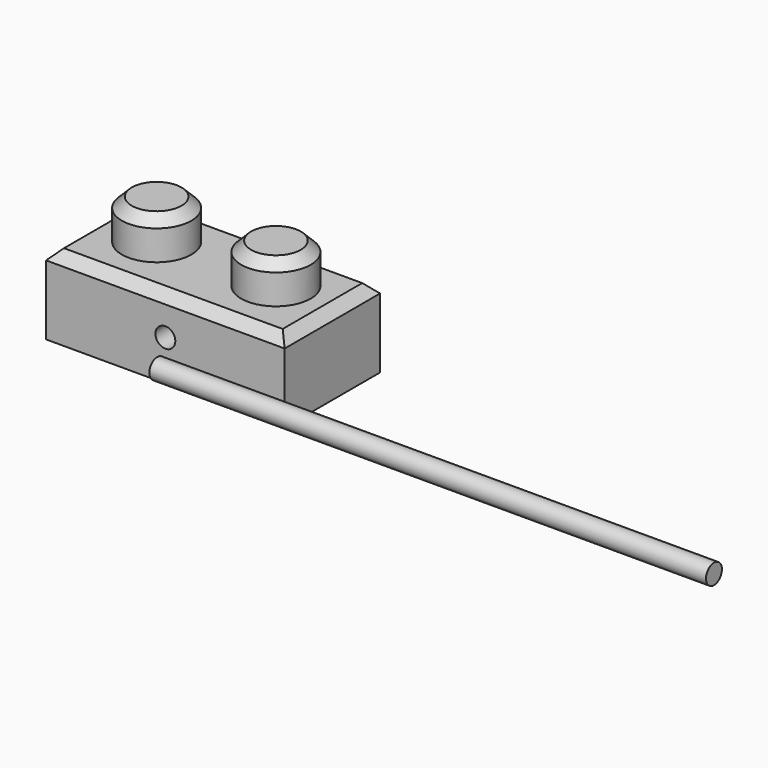
from build123d import *

# Parameters (mm, degrees)
F0_W          = 76.2
F0_H          = 38.1
F1_DEPTH      = 25.4
F2_R          = 11.1125
F3_DEPTH      = 12.7
F4_SIZE2      = 3.175
F4_SIZE       = 3.175
F5_SIZE       = 3.175
F6_T          = 7.9375
F7_R          = 3.175
F8_DEPTH      = 20.3260867754
F8_DEPTH_BACK = 17.7759132246
F9_R          = 3.175
F10_DEPTH     = 177.8


# Not quite as in the source:
# - a shell that OpenCascade refuses in one call is made with other operations: the cavity is built on its own and cut out


with BuildPart() as f1:
    # F0 (on Top) → F1 (new body)
    with BuildSketch(Plane.XY):
        with Locations((-14.6912483396, -1.2750867754)):
            Rectangle(F0_W, F0_H)
    extrude(amount=F1_DEPTH)

    # F2 (on face) → F3 (join)
    with BuildSketch(Plane.XY.offset(25.4)):
        with Locations((-33.7412483396, 0)):
            Circle(F2_R)
        with Locations((4.3587516604, 0)):
            Circle(F2_R)
    extrude(amount=F3_DEPTH)

    # F4
    f4_edges = [f1.edges().sort_by_distance(p)[0] for p in [
        (-14.691248, -20.325087, 25.4),
        (-52.791248, -1.275087, 25.4),
        (-14.691248, 17.774913, 25.4),
        (23.408752, -1.275087, 25.4),
    ]]
    chamfer(f4_edges, length=F4_SIZE, length2=F4_SIZE2)

    # F5
    f5_edges = [f1.edges().sort_by_distance(p)[0] for p in [
        (-44.853748, 0, 38.1),
        (-6.753748, 0, 38.1),
    ]]
    chamfer(f5_edges, length=F5_SIZE)

    # F6: shell of thickness 7.9375, made by hand


with BuildPart() as f6_core1:
    # F6_t2: copy of F1
    add(f1.part)

    # the walls: a layer under each face that stays
    f6_faces = [f6_core1.faces().sort_by_distance(p)[0] for p in [
        (-44.8537483396, 0, 30.1625),
        (-43.2662483396, 0, 36.5125),
        (-14.6912483396, -1.2750867754, 25.4),
        (-33.7412483396, 0, 38.1),
        (-14.6912483396, -18.7375867754, 23.8125),
        (-51.2037483396, -1.2750867754, 23.8125),
        (21.8212516604, -1.2750867754, 23.8125),
        (-14.6912483396, 16.1874132246, 23.8125),
        (-6.7537483396, 0, 30.1625),
        (-14.6912483396, -20.3250867754, 11.1125),
        (-52.7912483396, -1.2750867754, 11.1125),
        (23.4087516604, -1.2750867754, 11.1125),
        (-14.6912483396, 17.7749132246, 11.1125),
        (-5.1662483396, 0, 36.5125),
        (4.3587516604, 0, 38.1),
    ]]
    thicken(f6_faces, amount=-F6_T, mode=Mode.SUBTRACT)

    # F6_s3 → F6_t4 (revolve, cut)
    with BuildSketch(Plane.XZ):
        Polygon((-22.5493733396, 25.479375), (-30.5662483396, 25.4), (-30.5662483396, 17.4625), (-22.6287483396, 17.4625), align=None)
    revolve(axis=Axis((-33.7412483396, 0, 25.4), (0, 0, 1)), mode=Mode.SUBTRACT)

    # F6_s5 → F6_t6 (revolve, cut)
    with BuildSketch(Plane.XZ):
        Polygon((15.5506266604, 25.479375), (15.4712516604, 17.4625), (7.5337516604, 17.4625), (7.5337516604, 25.4), align=None)
    revolve(axis=Axis((4.3587516604, 0, 25.4), (0, 0, 1)), mode=Mode.SUBTRACT)


with BuildPart() as f1_1:
    add(f1.part)

    # what is left inside the walls is the cavity
    f6_cavity = [f6_core1.part.solids().sort_by_distance(p)[0] for p in [
        (-14.691248, -4.979253, 0.079375),
    ]]
    add(f6_cavity, mode=Mode.SUBTRACT)

    # F7 (on Front) → F8 (cut, two sides)
    with BuildSketch(Plane.XZ) as f8_sk:
        with Locations((-14.6912483396, 12.9471793771)):
            Circle(F7_R)
    extrude(amount=F8_DEPTH, mode=Mode.SUBTRACT)
    extrude(f8_sk.sketch, amount=-F8_DEPTH_BACK, mode=Mode.SUBTRACT)


with BuildPart() as f10:
    # F9 (on Right) → F10 (new body)
    with BuildSketch(Plane.YZ):
        with Locations((-41.9206805527, 17.8311616182)):
            Circle(F9_R)
    extrude(amount=F10_DEPTH)


solid = Compound([f1_1.part, f10.part])
